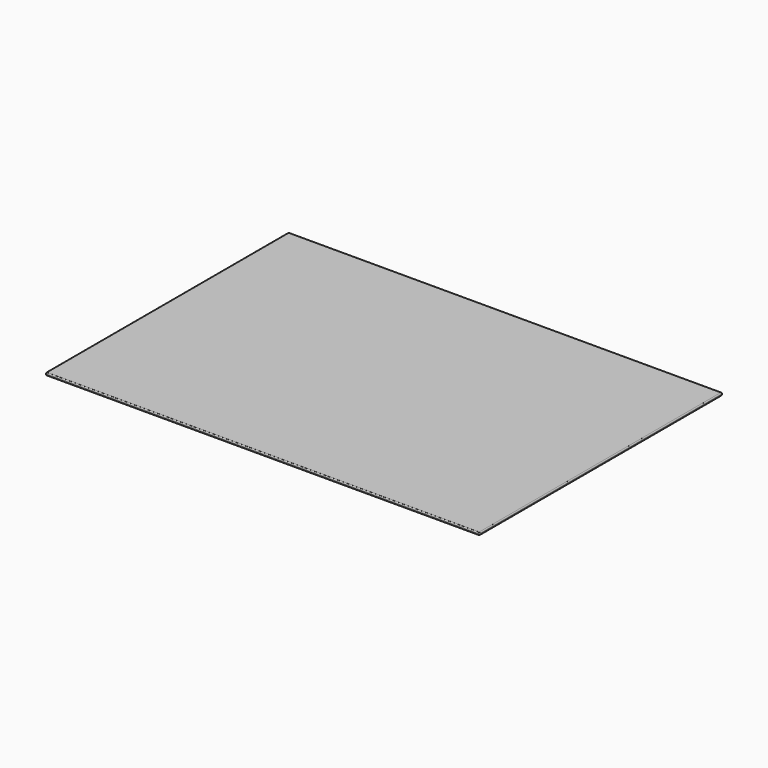
from build123d import *

# Parameters (mm, degrees)
F0_W         = 1000
F0_H         = 700
F1_DEPTH     = 6
F2_R         = 2
F3_R         = 2
F4_T1_DEPTH  = 696
F4_T3_DEPTH  = 2
F4_T5_DEPTH  = 996
F4_S9_W      = 2
F4_S9_H      = 2
F4_T10_DEPTH = 2
F4_S15_W     = 2
F4_S15_H     = 2
F4_T16_DEPTH = 2
F4_T20_ANGLE = 90
F4_T22_ANGLE = 90
F4_T24_ANGLE = 90
F4_T26_ANGLE = 90


# Not quite as in the source:
# - a fillet or chamfer that OpenCascade refuses, or shapes differently, is made with other operations: its cross-section is extruded or revolved along the edge and cut away or added


with BuildPart() as f1:
    # F0 (on Top) → F1 (new body)
    with BuildSketch(Plane.XY):
        with Locations((500, 350)):
            Rectangle(F0_W, F0_H)
    extrude(amount=F1_DEPTH)

    # F2
    f2_edges = [f1.edges().sort_by_distance(p)[0] for p in [
        (1000, 350, 0),
        (500, 700, 0),
        (500, 0, 6),
        (0, 350, 6),
    ]]
    fillet(f2_edges, radius=F2_R)

    # F3
    f3_edges = [f1.edges().sort_by_distance(p)[0] for p in [
        (499, 0, 0),
        (1000, 351, 6),
        (1000, 0, 3),
    ]]
    fillet(f3_edges, radius=F3_R)

    # F4: fillet of radius 2 on 2 edges, made by hand

    # F4_s2 → F4_t1 (cut)
    with BuildSketch(Plane.XZ.offset(-698)):
        with BuildLine():
            ThreePointArc((0, 2), (0.585786, 0.585786), (2, 0))
            Line((2, 0), (0, 0))
            Line((0, 0), (0, 2))
        make_face()
    extrude(amount=F4_T1_DEPTH, mode=Mode.SUBTRACT)

    # F4_s4 → F4_t3 (cut)
    with BuildSketch(Plane.XY.offset(2)):
        with BuildLine():
            ThreePointArc((0, 2), (0.585786, 0.585786), (2, 0))
            Line((2, 0), (0, 0))
            Line((0, 0), (0, 2))
        make_face()
        with BuildLine():
            ThreePointArc((0, 698), (0.585786, 699.414214), (2, 700))
            Line((2, 700), (0, 700))
            Line((0, 700), (0, 698))
        make_face()
        with BuildLine():
            ThreePointArc((998, 700), (999.414214, 699.414214), (1000, 698))
            Line((1000, 698), (1000, 700))
            Line((1000, 700), (998, 700))
        make_face()
    extrude(amount=F4_T3_DEPTH, mode=Mode.SUBTRACT)

    # F4_s6 → F4_t5 (cut)
    with BuildSketch(Plane.YZ.offset(2)):
        with BuildLine():
            ThreePointArc((700, 4), (699.414214, 5.414214), (698, 6))
            Line((698, 6), (700, 6))
            Line((700, 6), (700, 4))
        make_face()
    extrude(amount=F4_T5_DEPTH, mode=Mode.SUBTRACT)


with BuildPart() as f4_tool8:
    # F4_s9 → F4_t10 (new body)
    with BuildSketch(Plane.YZ.offset(2)):
        with Locations((1, 5)):
            Rectangle(F4_S9_W, F4_S9_H)
    extrude(amount=-F4_T10_DEPTH)

    # F4_s11 → F4_t12 (revolve, cut)
    with BuildSketch(Plane(origin=(2, 2, 4), x_dir=(0, 0.707107, -0.707107), z_dir=(0, 0.707107, 0.707107))):
        with BuildLine():
            ThreePointArc((0, -2), (2, 0), (0, 2))
            Line((0, 2), (0, -2))
        make_face()
    revolve(axis=Axis((2, 2, 4), (-1, 0, 0)), mode=Mode.SUBTRACT)


with BuildPart() as f1_1:
    add(f1.part)

    # F4_t7: cut F4_tool8
    add(f4_tool8.part, mode=Mode.SUBTRACT)


with BuildPart() as f4_tool14:
    # F4_s15 → F4_t16 (new body)
    with BuildSketch(Plane.XZ.offset(-698)):
        with Locations((999, 1)):
            Rectangle(F4_S15_W, F4_S15_H)
    extrude(amount=-F4_T16_DEPTH)

    # F4_s17 → F4_t18 (revolve, cut)
    with BuildSketch(Plane(origin=(998, 698, 2), x_dir=(-0.707107, 0, 0.707107), z_dir=(-0.707107, 0, -0.707107))):
        with BuildLine():
            ThreePointArc((0, -2), (2, 0), (0, 2))
            Line((0, 2), (0, -2))
        make_face()
    revolve(axis=Axis((998, 698, 2), (0, 1, 0)), mode=Mode.SUBTRACT)


with BuildPart() as f1_2:
    add(f1_1.part)

    # F4_t13: cut F4_tool14
    add(f4_tool14.part, mode=Mode.SUBTRACT)

    # F4_s19 → F4_t20 (revolve, cut)
    with BuildSketch(Plane.XZ.offset(-2)):
        with BuildLine():
            ThreePointArc((0, 2), (0.585786, 0.585786), (2, 0))
            Line((2, 0), (0, 0))
            Line((0, 0), (0, 2))
        make_face()
    revolve(axis=Axis((0, 2, 2), (-1, 0, 0)), revolution_arc=F4_T20_ANGLE, mode=Mode.SUBTRACT)

    # F4_s21 → F4_t22 (revolve, cut)
    with BuildSketch(Plane.XY.offset(2)):
        with BuildLine():
            ThreePointArc((0, 698), (0.585786, 699.414214), (2, 700))
            Line((2, 700), (0, 700))
            Line((0, 700), (0, 698))
        make_face()
    revolve(axis=Axis((0, 698, 2), (-1, 0, 0)), revolution_arc=F4_T22_ANGLE, mode=Mode.SUBTRACT)

    # F4_s23 → F4_t24 (revolve, cut)
    with BuildSketch(Plane.XY.offset(4)):
        with BuildLine():
            ThreePointArc((2, 700), (0.585786, 699.414214), (0, 698))
            Line((0, 698), (0, 700))
            Line((0, 700), (2, 700))
        make_face()
    revolve(axis=Axis((2, 700, 4), (0, 1, 0)), revolution_arc=F4_T24_ANGLE, mode=Mode.SUBTRACT)

    # F4_s25 → F4_t26 (revolve, cut)
    with BuildSketch(Plane.XY.offset(4)):
        with BuildLine():
            ThreePointArc((998, 700), (999.414214, 699.414214), (1000, 698))
            Line((1000, 698), (1000, 700))
            Line((1000, 700), (998, 700))
        make_face()
    revolve(axis=Axis((998, 700, 4), (0, -1, 0)), revolution_arc=F4_T26_ANGLE, mode=Mode.SUBTRACT)


solid = f1_2.part
